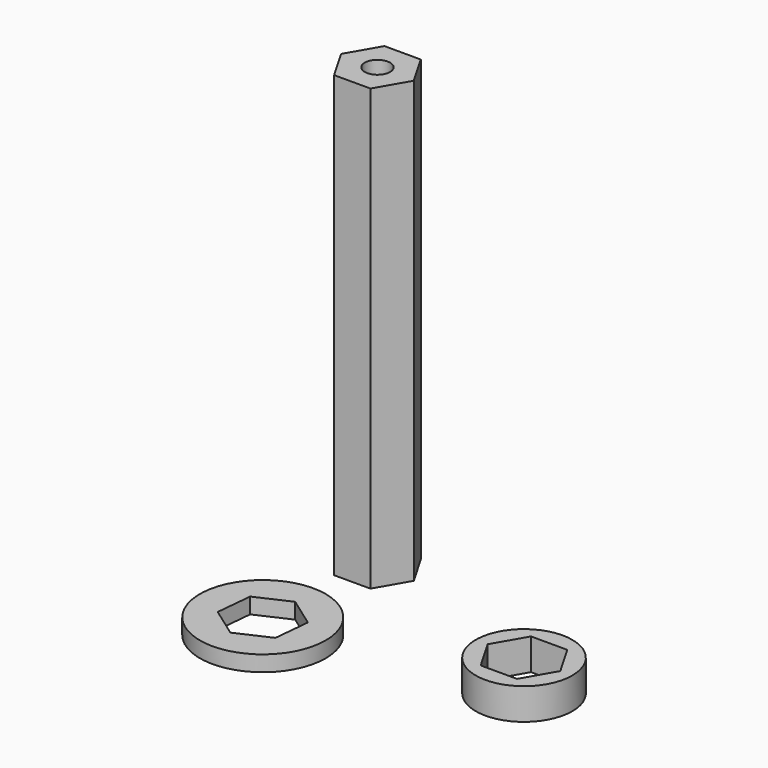
from build123d import *

# Parameters (mm, degrees)
F0_R     = 2.5527
F1_DEPTH = 88.9
F2_R     = 12.7
F3_DEPTH = 3.175
F4_R     = 9.7536
F5_DEPTH = 6.35


# Not quite as in the source:
# - a length typed as a fraction of an inch, garbled in the dataset ("3 / 203.2 mm" for 3/8 in), is restored


with BuildPart() as f1:
    # F0 (on Top) → F1 (new body)
    with BuildSketch(Plane.XY):
        Polygon((-65.3787461132, 30.7223642409), (-58.0463976945, 30.7223642409), (-54.3802234852, 37.0723642409), (-58.0463976945, 43.4223642409), (-65.3787461132, 43.4223642409), (-69.0449203226, 37.0723642409), align=None)
        with Locations((-61.7125719039, 37.0723642409)):
            Circle(F0_R, mode=Mode.SUBTRACT)
    extrude(amount=F1_DEPTH)


with BuildPart() as f3:
    # F2 (on Top) → F3 (new body)
    with BuildSketch(Plane.XY):
        with Locations((-61.4009574056, 7.7439234592)):
            Circle(F2_R)
        Polygon((-54.7258350544, 10.7780748942), (-55.4357440084, 3.4801736472), (-62.1108663595, 0.4460222122), (-68.0760797567, 4.7097720242), (-67.3661708028, 12.0076732712), (-60.6910484516, 15.0418247062), align=None, mode=Mode.SUBTRACT)
    extrude(amount=F3_DEPTH)


with BuildPart() as f5:
    # F4 (on Top) → F5 (new body)
    with BuildSketch(Plane.XY):
        with Locations((-16.8024227023, 17.9264470935)):
            Circle(F4_R)
        Polygon((-9.4700742836, 17.9264470935), (-13.136248493, 11.5764470935), (-20.4685969117, 11.5764470935), (-24.134771121, 17.9264470935), (-20.4685969117, 24.2764470935), (-13.136248493, 24.2764470935), align=None, mode=Mode.SUBTRACT)
    extrude(amount=F5_DEPTH)


solid = Compound([f1.part, f3.part, f5.part])
